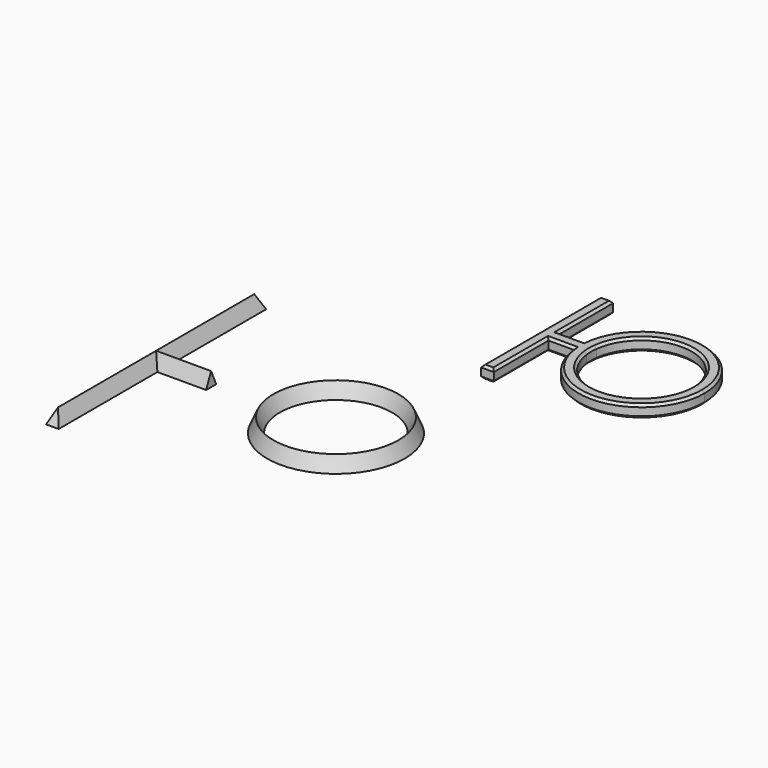
from build123d import *

# Parameters (mm, degrees)
F0_R       = 17.5
F0_R_2     = 14.3
F1_DEPTH   = 3.6
F0_W       = 1.6
F0_H       = 3.2
F0_W_2     = 12.4
F2_SIZE2   = 1.59999
F2_SIZE    = 3.59999
F2_2_SIZE2 = 1.59999
F2_2_SIZE  = 3.59999
F3_SIZE2   = 3.59999
F3_SIZE    = 1.79999
F4_SIZE2   = 3.59999
F4_SIZE    = 1.59999
F5_W       = 1.6
F5_H       = 3.2
F6_DEPTH   = 3.2
F7_SIZE    = 0.6


# Not quite as in the source:
# - a fillet or chamfer is up to 0.001 mm smaller than in the source, because OpenCascade refuses the exact size


with BuildPart() as f1:
    # F0 (on Top) → F1 (new body)
    with BuildSketch(Plane.XY):
        Circle(F0_R)
        Circle(F0_R_2, mode=Mode.SUBTRACT)
    extrude(amount=F1_DEPTH)

    # F2 (size 3.6 and 1.6 in the source; OpenCascade refuses exactly that, so slightly less here)
    f2_edges = [f1.edges().sort_by_distance(p)[0] for p in [
        (-14.3, 0, 3.6),
    ]]
    f2_side = f1.faces().sort_by_distance((-14.3, 0, 1.8))[0]
    chamfer(f2_edges, length=F2_SIZE, length2=F2_SIZE2, reference=f2_side)

    # F2#2 (size 3.6 and 1.6 in the source; OpenCascade refuses exactly that, so slightly less here)
    f2_2_edges = [f1.edges().sort_by_distance(p)[0] for p in [
        (-17.5, 0, 3.6),
    ]]
    f2_2_side = f1.faces().sort_by_distance((-17.5, 0, 1.8))[0]
    chamfer(f2_2_edges, length=F2_2_SIZE, length2=F2_2_SIZE2, reference=f2_2_side)


with BuildPart() as f1b:
    # F0 (on Top) → F1, piece 2 (new body)
    with BuildSketch(Plane.XY):
        Polygon((-45.7531064749, -1.6), (-45.7531064749, 1.6), (-44.1531064749, 1.6), (-44.1531064749, 33), (-47.3531064749, 33), (-47.3531064749, -33), (-44.1531064749, -33), (-44.1531064749, -1.6), align=None)
        with Locations((-44.9531064749, 0)):
            Rectangle(F0_W, F0_H)
        with Locations((-37.9531064749, 0)):
            Rectangle(F0_W_2, F0_H)
    extrude(amount=F1_DEPTH)

    # F3 (size 1.8 and 3.6 in the source; OpenCascade refuses exactly that, so slightly less here)
    f3_edges = [f1b.edges().sort_by_distance(p)[0] for p in [
        (-45.753106, -33, 3.6),
        (-45.753106, 33, 3.6),
    ]]
    f3_side = f1b.faces().sort_by_distance((-44.519433, 0, 3.6))[0]
    chamfer(f3_edges, length=F3_SIZE, length2=F3_SIZE2, reference=f3_side)

    # F4 (size 1.6 and 3.6 in the source; OpenCascade refuses exactly that, so slightly less here)
    f4_edges = [f1b.edges().sort_by_distance(p)[0] for p in [
        (-47.353106, 0, 3.6),
        (-44.153106, 16.400005, 3.6),
        (-44.153106, -16.400005, 3.6),
        (-37.953106, -1.6, 3.6),
        (-37.953106, 1.6, 3.6),
    ]]
    f4_side = f1b.faces().sort_by_distance((-44.460059, 0, 3.6))[0]
    chamfer(f4_edges, length=F4_SIZE, length2=F4_SIZE2, reference=f4_side)


with BuildPart() as f6:
    # F5 (on Top) → F6 (new body)
    with BuildSketch(Plane.XY):
        with BuildLine():
            ThreePointArc((17.6622043613, 53.6302412689), (34.383007756, 39.2503040991), (49.582003355, 55.2302412689))
            ThreePointArc((49.582003355, 55.2302412689), (34.383007756, 71.2101784386), (17.6622043613, 56.8302412689))
            Line((17.6622043613, 56.8302412689), (20.8823970619, 56.8302412689))
            ThreePointArc((20.8823970619, 56.8302412689), (34.3835766356, 68.0051181871), (46.382003355, 55.2302412689))
            ThreePointArc((46.382003355, 55.2302412689), (34.3835766356, 42.4553643506), (20.8823970619, 53.6302412689))
            Line((20.8823970619, 53.6302412689), (17.6622043613, 53.6302412689))
        make_face()
        with BuildLine():
            Line((20.8823970619, 56.8302412689), (17.6622043613, 56.8302412689))
            ThreePointArc((17.6622043613, 56.8302412689), (17.582003355, 55.2302412689), (17.6622043613, 53.6302412689))
            Line((17.6622043613, 53.6302412689), (20.8823970619, 53.6302412689))
            ThreePointArc((20.8823970619, 53.6302412689), (20.782003355, 55.2302412689), (20.8823970619, 56.8302412689))
        make_face()
        with BuildLine():
            ThreePointArc((17.6622043613, 53.6302412689), (17.582003355, 55.2302412689), (17.6622043613, 56.8302412689))
            Line((17.6622043613, 56.8302412689), (11.182003355, 56.8302412689))
            Line((11.182003355, 56.8302412689), (11.182003355, 53.6302412689))
            Line((11.182003355, 53.6302412689), (17.6622043613, 53.6302412689))
        make_face()
        with Locations((10.382003355, 55.2302412689)):
            Rectangle(F5_W, F5_H)
        Polygon((9.582003355, 56.8302412689), (11.182003355, 56.8302412689), (11.182003355, 74.2302412689), (7.982003355, 74.2302412689), (7.982003355, 36.2302412689), (11.182003355, 36.2302412689), (11.182003355, 53.6302412689), (9.582003355, 53.6302412689), align=None)
    extrude(amount=F6_DEPTH)

    # F7
    f7_edges = [f6.edges().sort_by_distance(p)[0] for p in [
        (14.422104, 56.830241, 3.2),
        (11.182003, 65.530241, 3.2),
        (9.582003, 74.230241, 3.2),
        (7.982003, 55.230241, 3.2),
        (9.582003, 36.230241, 3.2),
        (11.182003, 44.930241, 3.2),
        (14.422104, 53.630241, 3.2),
        (49.582003, 55.230241, 3.2),
        (20.782003, 55.230241, 3.2),
        (14.422104, 56.830241, 0),
        (11.182003, 65.530241, 0),
        (9.582003, 74.230241, 0),
        (7.982003, 55.230241, 0),
        (9.582003, 36.230241, 0),
        (11.182003, 44.930241, 0),
        (14.422104, 53.630241, 0),
        (49.582003, 55.230241, 0),
        (20.782003, 55.230241, 0),
    ]]
    chamfer(f7_edges, length=F7_SIZE)


solid = Compound([f1.part, f1b.part, f6.part])
